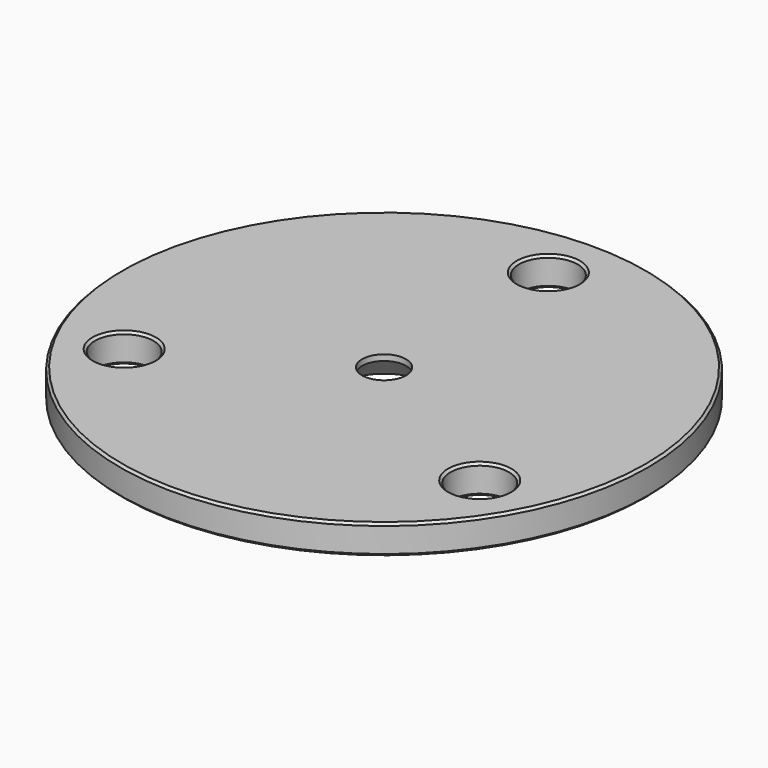
from build123d import *

# Parameters (mm, degrees)
F0_R     = 57.15
F0_R_2   = 6.35
F0_R_3   = 4.7625
F1_DEPTH = 6.35
F2_SIZE  = 0.508
F3_SIZE  = 5.08


# Not quite as in the source:
# - a feature names something its author has since deleted; it is built from what else it names


with BuildPart() as f1:
    # F0 (on Top) → F1 (new body)
    with BuildSketch(Plane.XY):
        Circle(F0_R)
        with Locations((-38.4948291982, -22.225)):
            Circle(F0_R_2, mode=Mode.SUBTRACT)
        with Locations((38.4948291982, -22.225)):
            Circle(F0_R_2, mode=Mode.SUBTRACT)
        Circle(F0_R_3, mode=Mode.SUBTRACT)
        with Locations((0, 44.45)):
            Circle(F0_R_2, mode=Mode.SUBTRACT)
    extrude(amount=F1_DEPTH)

    # F2
    f2_edges = [f1.edges().sort_by_distance(p)[0] for p in [
        (-57.15, 0, 6.35),
        (-6.35, 44.45, 6.35),
        (-44.844829, -22.225, 6.35),
        (32.144829, -22.225, 6.35),
        (-57.15, 0, 0),
        (-6.35, 44.45, 0),
        (32.144829, -22.225, 0),
        (-44.844829, -22.225, 0),
    ]]
    chamfer(f2_edges, length=F2_SIZE)

    # F3
    f3_edges = [f1.edges().sort_by_distance(p)[0] for p in [
        (-4.7625, 0, 0),
    ]]
    chamfer(f3_edges, length=F3_SIZE)


solid = f1.part
